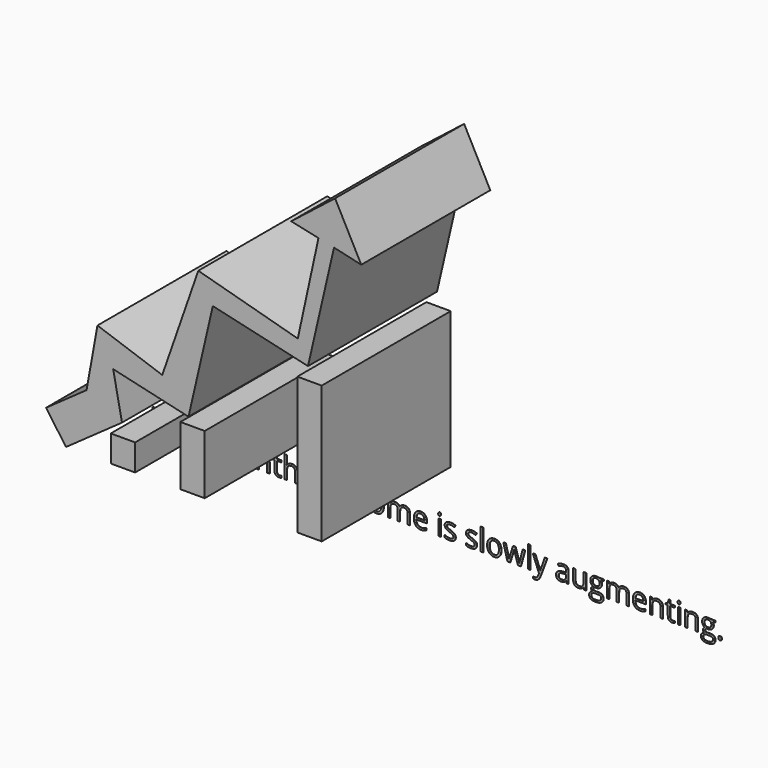
from build123d import *

# Parameters (mm, degrees)
F1_DEPTH     = 25.4
F0_W         = 3.8366322406
F0_H         = 9.3293590471
F0_H_2       = 4.1773109697
F0_H_3       = 21.606579423
F2_TEXT_SIZE = 4.5461664235
F3_DEPTH     = 0.0508


# Not quite as in the source:
# - Text() gives the source's letters only with a copy of the font that has no kerning and outlines rounded to 1/6400 em; it was checked with that copy


with BuildPart() as f1:
    # F0 (on Front) → F1 (new body)
    with BuildSketch(Plane.XZ):
        Polygon((-3.1340324786, 4.4245161116), (0, 0), (8.8182737829, 6.246277727), (7.4337245896, 13.2159059867), (19.2963555455, 10.4783764109), (23.1236232404, 27.0632069949), (38.1090004781, 23.6050438314), (42.2109003048, 41.3799472669), (40.9867731323, 41.6373666634), (39.7626459599, 41.8947860599), (36.503687501, 26.9035547972), (20.8351196231, 31.2142810254), (15.1574695483, 14.9105666205), (4.9569117837, 18.4628367424), (3.2401311898, 8.9395490455), align=None)
        Polygon((35.4655233586, 42.8289417543), (39.7626459599, 41.8947860599), (40.9867731323, 41.6373666634), (42.3780803698, 48.2535619388), align=None)
        Polygon((40.9867731323, 41.6373666634), (42.2109003048, 41.3799472669), (46.4957749213, 40.3911302806), (42.3780803698, 48.2535619388), align=None)
    extrude(amount=F1_DEPTH)


with BuildPart() as f1b:
    # F0 (on Front) → F1, piece 2 (new body)
    with BuildSketch(Plane.XZ):
        with Locations((19.9323317502, 4.6646795236)):
            Rectangle(F0_W, F0_H)
    extrude(amount=F1_DEPTH)


with BuildPart() as f1c:
    # F0 (on Front) → F1, piece 3 (new body)
    with BuildSketch(Plane.XZ):
        with Locations((8.9705276769, 2.0886554848)):
            Rectangle(F0_W, F0_H_2)
    extrude(amount=F1_DEPTH)


with BuildPart() as f1d:
    # F0 (on Front) → F1, piece 4 (new body)
    with BuildSketch(Plane.XZ):
        with Locations((38.3481646422, 10.8032897115)):
            Rectangle(F0_W, F0_H_3)
    extrude(amount=F1_DEPTH)


with BuildPart() as f3:
    # F2 (on Front) → F3 (new body)
    with BuildSketch(Plane.XZ):
        with Locations((-6.666678004, -10.1668937132)):
            Text('The monthly income is slowly augmenting.', F2_TEXT_SIZE, font='Open Sans', text_align=(TextAlign.LEFT, TextAlign.BOTTOM))
    extrude(amount=F3_DEPTH)


solid = Compound([f1.part, f1b.part, f1c.part, f1d.part, f3.part])
